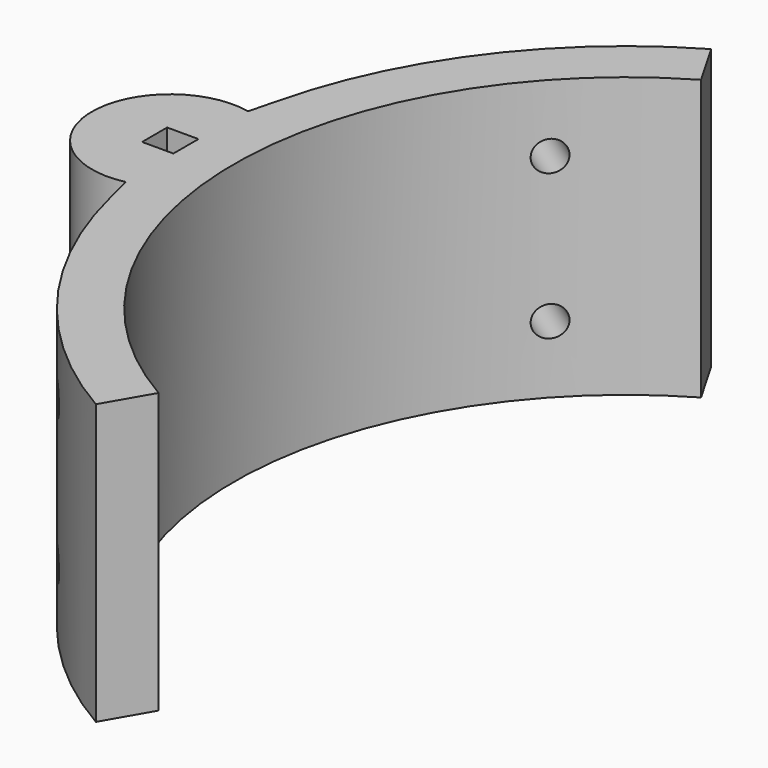
from build123d import *

# Parameters (mm, degrees)
F0_R     = 1.27
F1_DEPTH = 15.875
F2_W     = 3.556
F2_H     = 3.556
F3_DEPTH = 31.751
F6_D     = 3.4544


# Not quite as in the source:
# - a pattern or mirror of a feature is missing from the dataset's text; its kind, count and spacing are read off the source's solid


with BuildPart() as f1:
    # F0 (on Top) → F1 (new body, symmetric)
    with BuildSketch(Plane.XY):
        with BuildLine():
            ThreePointArc((-22.225, -38.4948291982), (-44.45, 0), (-22.225, 38.4948291982))
            Line((-22.225, 38.4948291982), (-25.2095, 43.6641348334))
            ThreePointArc((-25.2095, 43.6641348334), (-40.4033060907, 30.1603782792), (-49.0297327529, 11.7541850921))
            Line((-49.0297327529, 11.7541850921), (-49.807311051, 8.6885756427))
            ThreePointArc((-49.807311051, 8.6885756427), (-60.579, 0), (-49.807311051, -8.6885756427))
            Line((-49.807311051, -8.6885756427), (-49.0297327529, -11.7541850921))
            ThreePointArc((-49.0297327529, -11.7541850921), (-40.4033060907, -30.1603782792), (-25.2095, -43.6641348334))
            Line((-25.2095, -43.6641348334), (-22.225, -38.4948291982))
        make_face()
        with Locations((-51.689, 0)):
            Circle(F0_R, mode=Mode.SUBTRACT)
    extrude(amount=F1_DEPTH, both=True)

    # F2 (on face) → F3 (cut, through all)
    with BuildSketch(Plane.XY.offset(15.875)):
        with Locations((-51.689, 0)):
            Rectangle(F2_W, F2_H)
    extrude(amount=-F3_DEPTH, mode=Mode.SUBTRACT)

    # F6 (through all)
    with Locations(Plane(origin=(-33.0630224343, 22.7295389308, 0), x_dir=(-0.5665070073, -0.824056922, 0), z_dir=(0.824056922, -0.5665070073, 0))):
        with Locations((-6.3126659952, -8.255), (-6.3126659952, 8.255)):
            f6 = Hole(F6_D / 2)

    # F6_copies: F6 across plane
    add(f6.mirror(Plane(origin=(0, -4.4e-05, 0), x_dir=(-1, 1e-06, 0), z_dir=(-1e-06, -1, 0))), mode=Mode.SUBTRACT)


solid = f1.part
